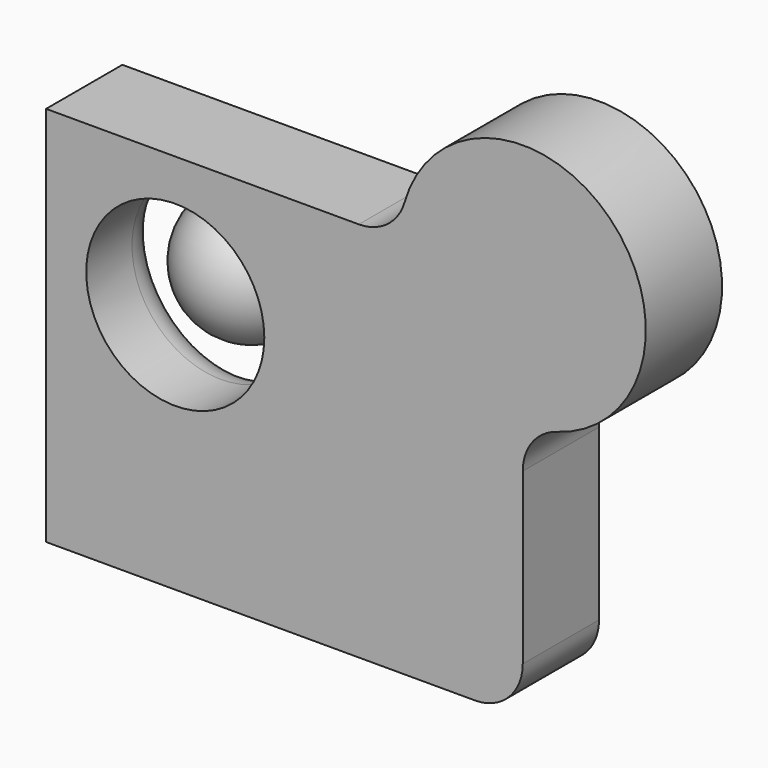
from build123d import *

# Parameters (mm, degrees)
F0_R        = 11.8611520112
F1_DEPTH    = 12.7
F4_R        = 5.08
F5_W        = 22.3380420357
F5_H        = 10.8657181263
F6_DEPTH    = 2.54
F7_T1_DEPTH = 21.8642407544
F8_T1_DEPTH = 10.8657181263


# Not quite as in the source:
# - a fillet or chamfer that OpenCascade refuses, or shapes differently, is made with other operations: its cross-section is extruded or revolved along the edge and cut away or added


with BuildPart() as f1:
    # F0 (on Front) → F1 (new body)
    with BuildSketch(Plane.XZ):
        with BuildLine():
            Line((7.4144873275, 31.8395160139), (-34.2452449948, 31.8395160139))
            Line((-34.2452449948, 31.8395160139), (-34.2452449948, -18.9604839861))
            Line((-34.2452449948, -18.9604839861), (22.9047550052, -18.9604839861))
            ThreePointArc((22.9047550052, -18.9604839861), (27.3948830658, -17.1006120467), (29.2547550052, -12.6104839861))
            Line((29.2547550052, -12.6104839861), (29.2547550052, 9.9992483361))
            ThreePointArc((29.2547550052, 9.9992483361), (30.5263698523, 13.8114005154), (33.8319216944, 16.0967529119))
            ThreePointArc((33.8319216944, 16.0967529119), (40.8475338995, 43.4322949081), (13.5119919033, 36.416682703))
            ThreePointArc((13.5119919033, 36.416682703), (11.2266395068, 33.1111308609), (7.4144873275, 31.8395160139))
        make_face()
        with Locations((-17.0359034091, 14.4511451945)):
            Circle(F0_R, mode=Mode.SUBTRACT)
    extrude(amount=F1_DEPTH)

    # F4
    f4_edges = [f1.edges().sort_by_distance(p)[0] for p in [
        (-28.897055, 0, 14.451145),
    ]]
    fillet(f4_edges, radius=F4_R)

    # F5 (on face) → F6 (cut)
    with BuildSketch(Plane(origin=(0, 0, 0), x_dir=(-1, 0, 0), z_dir=(0, 1, 0))):
        with Locations((-29.3970992789, 32.0457555354)):
            Rectangle(F5_W, F5_H)
        with BuildLine():
            Line((-33.1119049952, 35.6353998723), (-33.1119049952, 28.6111626774))
            Line((-33.1119049952, 28.6111626774), (-33.9282477289, 28.6111626774))
            Line((-33.9282477289, 28.6111626774), (-33.9282477289, 31.5137146196))
            add(Edge.make_bspline(
                [(-33.9282477289, 31.5137146196), (-34.6446615028, 31.2585114298), (-35.1204770886, 31.1647319443)],
                knots=[0, 0, 0, 1, 1, 1], degree=2))
            add(Edge.make_bspline(
                [(-35.1204770886, 31.1647319443), (-35.5962926745, 31.0709524589), (-36.1051616856, 31.0709524589)],
                knots=[0, 0, 0, 1, 1, 1], degree=2))
            add(Edge.make_bspline(
                [(-36.1051616856, 31.0709524589), (-37.0998391785, 31.0709524589), (-37.6356121402, 31.5275509371)],
                knots=[0, 0, 0, 1, 1, 1], degree=2))
            add(Edge.make_bspline(
                [(-37.6356121402, 31.5275509371), (-38.171385102, 31.9841494153), (-38.171385102, 32.8435384702)],
                knots=[0, 0, 0, 1, 1, 1], degree=2))
            Line((-38.171385102, 32.8435384702), (-38.171385102, 35.6353998723))
            Line((-38.171385102, 35.6353998723), (-37.3535049997, 35.6353998723))
            Line((-37.3535049997, 35.6353998723), (-37.3535049997, 32.9403926929))
            add(Edge.make_bspline(
                [(-37.3535049997, 32.9403926929), (-37.3535049997, 32.359267357), (-37.0491060142, 32.0802349537)],
                knots=[0, 0, 0, 1, 1, 1], degree=2))
            add(Edge.make_bspline(
                [(-37.0491060142, 32.0802349537), (-36.7447070287, 31.8012025503), (-36.0575032585, 31.8012025503)],
                knots=[0, 0, 0, 1, 1, 1], degree=2))
            add(Edge.make_bspline(
                [(-36.0575032585, 31.8012025503), (-35.5916805687, 31.8012025503), (-35.1658294627, 31.8711528222)],
                knots=[0, 0, 0, 1, 1, 1], degree=2))
            add(Edge.make_bspline(
                [(-35.1658294627, 31.8711528222), (-34.7399783568, 31.9411030941), (-33.9282477289, 32.2055304957)],
                knots=[0, 0, 0, 1, 1, 1], degree=2))
            Line((-33.9282477289, 32.2055304957), (-33.9282477289, 35.6353998723))
            Line((-33.9282477289, 35.6353998723), (-33.1119049952, 35.6353998723))
        make_face(mode=Mode.SUBTRACT)
        Polygon((-31.1855821225, 35.6353998723), (-27.2699042641, 35.6353998723), (-27.2699042641, 34.900537675), (-30.3692393888, 34.900537675), (-30.3692393888, 28.6111626774), (-31.1855821225, 28.6111626774), align=None, mode=Mode.SUBTRACT)
        Polygon((-24.2581991503, 32.223978919), (-21.0143513759, 28.6111626774), (-22.004416763, 28.6111626774), (-25.2528766432, 32.1717083862), (-25.2528766432, 28.6111626774), (-26.0692193769, 28.6111626774), (-26.0692193769, 35.6353998723), (-25.2528766432, 35.6353998723), (-25.2528766432, 32.2332031307), (-22.0858972995, 35.6353998723), (-21.1496398139, 35.6353998723), align=None, mode=Mode.SUBTRACT)
    extrude(amount=-F6_DEPTH, mode=Mode.SUBTRACT)

    # F7: fillet of radius 5.08 on 1 edges, made by hand

    # F7_s2 → F7_t1 (join)
    with BuildSketch(Plane.XY.offset(15.6143738442)):
        with BuildLine():
            ThreePointArc((18.228078261, 0), (20.0874873122, -1.8594090512), (22.6274873122, -2.54))
            Line((22.6274873122, -2.54), (18.228078261, -2.54))
            Line((18.228078261, -2.54), (18.228078261, 0))
        make_face()
    extrude(amount=F7_T1_DEPTH)

    # F8: fillet of radius 5.08 on 1 edges, made by hand

    # F8_s2 → F8_t1 (join)
    with BuildSketch(Plane.XY.offset(26.6128964722)):
        with BuildLine():
            ThreePointArc((40.5661202967, 0), (38.7067112455, -1.8594090512), (36.1667112455, -2.54))
            Line((36.1667112455, -2.54), (40.5661202967, -2.54))
            Line((40.5661202967, -2.54), (40.5661202967, 0))
        make_face()
    extrude(amount=F8_T1_DEPTH)


with BuildPart() as f3:
    # F2 (on face) → F3 (revolve)
    with BuildSketch(Plane(origin=(0, 0, 0), x_dir=(-1, 0, 0), z_dir=(0, 1, 0))):
        with BuildLine():
            Line((17.0359034091, 14.4511451945), (17.0359034091, 23.2243563161))
            ThreePointArc((17.0359034091, 23.2243563161), (8.2626922875, 14.4511451945), (17.0359034091, 5.6779340729))
            Line((17.0359034091, 5.6779340729), (17.0359034091, 14.4511451945))
        make_face()
    revolve(axis=Axis((-17.0359034091, 0, 14.4511451945), (0, 0, -1)))


solid = Compound([f1.part, f3.part])
